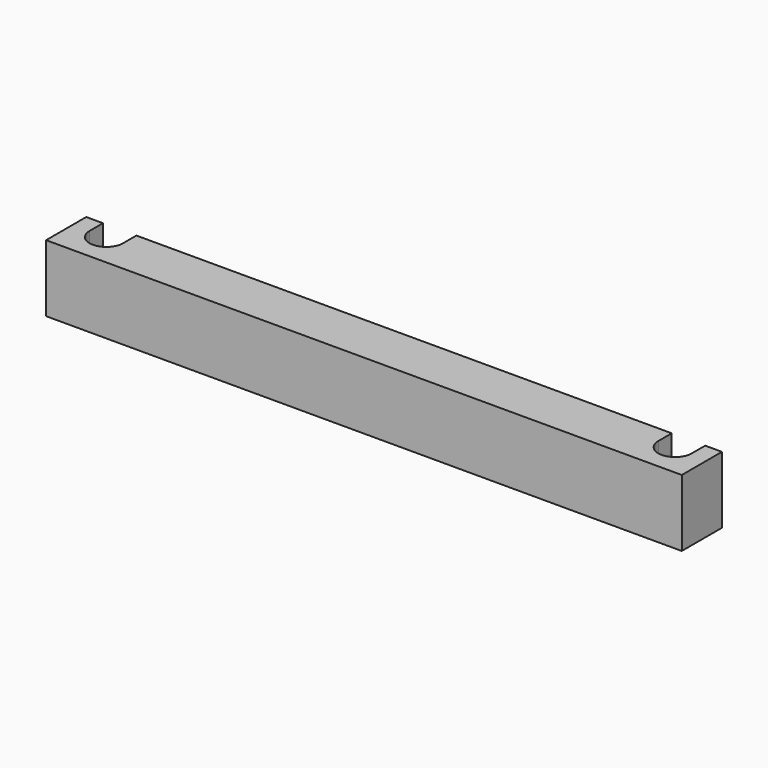
from build123d import *

# Parameters (mm, degrees)
F1_DEPTH = 20
F2_DEPTH = 5


with BuildPart() as f1:
    # F0 (on Top) → F1 (new body)
    with BuildSketch(Plane.XY):
        with BuildLine():
            Line((54.1798012435, 12.6796376905), (-105.8201987565, 12.6796376905))
            ThreePointArc((-105.8201987565, 12.6796376905), (-110.8201987565, 7.6796376905), (-115.8201987565, 12.6796376905))
            Line((-115.8201987565, 12.6796376905), (-120.8201987565, 12.6796376905))
            Line((-120.8201987565, 12.6796376905), (-120.8201987565, 2.6796376905))
            Line((-120.8201987565, 2.6796376905), (69.1798012435, 2.6796376905))
            Line((69.1798012435, 2.6796376905), (69.1798012435, 12.6796376905))
            Line((69.1798012435, 12.6796376905), (64.1798012435, 12.6796376905))
            ThreePointArc((64.1798012435, 12.6796376905), (59.1798012435, 7.6796376905), (54.1798012435, 12.6796376905))
        make_face()
    extrude(amount=F1_DEPTH)

    # F2 (add): faces of the model
    f2_faces = [f1.faces().sort_by_distance(p)[0] for p in [
        (-25.8201987565, 12.6796376905, 10),
        (-118.3201987565, 12.6796376905, 10),
        (66.6798012435, 12.6796376905, 10),
    ]]
    extrude(f2_faces, amount=F2_DEPTH)


solid = f1.part
